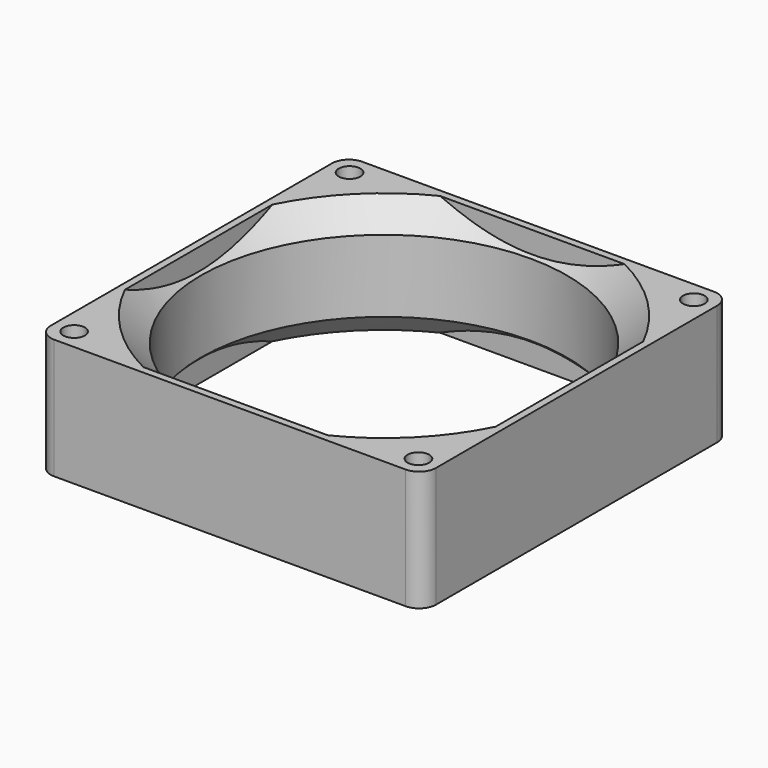
from build123d import *

# Parameters (mm, degrees)
F0_R     = 2.25
F0_R_2   = 38
F1_DEPTH = 25
F3_W     = 1.5
F3_H     = 38.3014360044
F3_W_2   = 38.3014360044
F3_H_2   = 1.5
F4_DEPTH = 25


# Not quite as in the source:
# - a fillet or chamfer that OpenCascade refuses, or shapes differently, is made with other operations: its cross-section is extruded or revolved along the edge and cut away or added


with BuildPart() as f1:
    # F0 (on Top) → F1 (new body)
    with BuildSketch(Plane.XY):
        with BuildLine():
            Line((-36.5, -40), (36.5, -40))
            ThreePointArc((36.5, -40), (38.9748737342, -38.9748737342), (40, -36.5))
            Line((40, -36.5), (40, 36.5))
            ThreePointArc((40, 36.5), (38.9748737342, 38.9748737342), (36.5, 40))
            Line((36.5, 40), (-36.5, 40))
            ThreePointArc((-36.5, 40), (-38.9748737342, 38.9748737342), (-40, 36.5))
            Line((-40, 36.5), (-40, -36.5))
            ThreePointArc((-40, -36.5), (-38.9748737342, -38.9748737342), (-36.5, -40))
        make_face()
        with Locations((-35.75, -35.75)):
            Circle(F0_R, mode=Mode.SUBTRACT)
        with Locations((35.75, -35.75)):
            Circle(F0_R, mode=Mode.SUBTRACT)
        with Locations((-35.75, 35.75)):
            Circle(F0_R, mode=Mode.SUBTRACT)
        Circle(F0_R_2, mode=Mode.SUBTRACT)
        with Locations((35.75, 35.75)):
            Circle(F0_R, mode=Mode.SUBTRACT)
    extrude(amount=F1_DEPTH)

    # F2: chamfer of 5 on 2 edges, made by hand

    # F2_s1 → F2_t2 (revolve, cut)
    with BuildSketch(Plane.XZ):
        Polygon((38, 20), (43, 25), (38, 25), align=None)
    revolve(axis=Axis((0, 0, 25), (0, 0, 1)), mode=Mode.SUBTRACT)

    # F2_s3 → F2_t4 (revolve, cut)
    with BuildSketch(Plane.XZ):
        Polygon((38, 5), (43, 0), (38, 0), align=None)
    revolve(axis=Axis((0, 0, 0), (0, 0, 1)), mode=Mode.SUBTRACT)

    # F3 (on face) → F4 (join, through all)
    with BuildSketch(Plane.XY.offset(25)):
        with Locations((-39.25, 0)):
            Rectangle(F3_W, F3_H)
        with Locations((0, -39.25)):
            Rectangle(F3_W_2, F3_H_2)
        with Locations((39.25, 0)):
            Rectangle(F3_W, F3_H)
        with Locations((0, 39.25)):
            Rectangle(F3_W_2, F3_H_2)
    extrude(amount=-F4_DEPTH)


solid = f1.part
